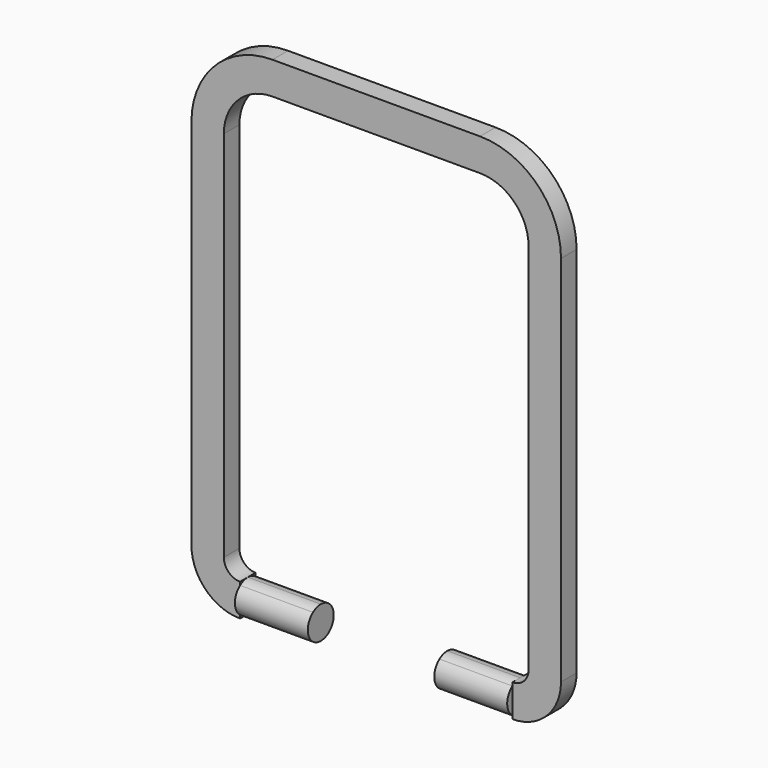
from build123d import *
from build123d import SkipClean  # not in build123d's __all__

# Parameters (mm, degrees)
F1_DEPTH = 1.2
F3_DEPTH = 4.5
F4_DEPTH = 4.5
F6_DEPTH = 4.5
F7_DEPTH = 4.5


with BuildPart() as f1:
    # F0 (on Front) → F1 (new body)
    with BuildSketch(Plane.XZ):
        with BuildLine():
            Line((5.55, 0), (-7.25, 0))
            ThreePointArc((-7.25, 0), (-10.7855339059, -1.4644660941), (-12.25, -5))
            Line((-12.25, -5), (-12.25, -28))
            ThreePointArc((-12.25, -28), (-11.3713203436, -30.1213203436), (-9.25, -31))
            Line((-9.25, -31), (-4.75, -31))
            Line((-4.75, -31), (-4.75, -29))
            Line((-4.75, -29), (-9.25, -29))
            ThreePointArc((-9.25, -29), (-9.9571067812, -28.7071067812), (-10.25, -28))
            Line((-10.25, -28), (-10.25, -5))
            ThreePointArc((-10.25, -5), (-9.3713203436, -2.8786796564), (-7.25, -2))
            Line((-7.25, -2), (5.55, -2))
            ThreePointArc((5.55, -2), (7.6713203436, -2.8786796564), (8.55, -5))
            Line((8.55, -5), (8.55, -28))
            ThreePointArc((8.55, -28), (8.2571067812, -28.7071067812), (7.55, -29))
            Line((7.55, -29), (3.05, -29))
            Line((3.05, -29), (3.05, -31))
            Line((3.05, -31), (7.55, -31))
            ThreePointArc((7.55, -31), (9.6713203436, -30.1213203436), (10.55, -28))
            Line((10.55, -28), (10.55, -5))
            ThreePointArc((10.55, -5), (9.0855339059, -1.4644660941), (5.55, 0))
        make_face()
    extrude(amount=F1_DEPTH)

    # F2 (on face) → F3 (join)
    with BuildSketch(Plane.YZ.offset(-4.75)):
        with BuildLine():
            Line((-1.2, -30.8), (-1.2, -29.2))
            ThreePointArc((-1.2, -29.2), (-1.6, -30), (-1.2, -30.8))
        make_face()
        with BuildLine():
            ThreePointArc((-0.6, -29), (-0.916227766, -29.0513167019), (-1.2, -29.2))
            Line((-1.2, -29.2), (-1.2, -30.8))
            ThreePointArc((-1.2, -30.8), (-0.916227766, -30.9486832981), (-0.6, -31))
            ThreePointArc((-0.6, -31), (-0.283772234, -30.9486832981), (0, -30.8))
            Line((0, -30.8), (0, -29.2))
            ThreePointArc((0, -29.2), (-0.283772234, -29.0513167019), (-0.6, -29))
        make_face()
        with BuildLine():
            ThreePointArc((0.4, -30), (0.294427191, -29.5527864045), (0, -29.2))
            Line((0, -29.2), (0, -30.8))
            ThreePointArc((0, -30.8), (0.294427191, -30.4472135955), (0.4, -30))
        make_face()
    extrude(amount=-F3_DEPTH)

    # F2 (on face) → F4 (cut)
    with BuildSketch(Plane.YZ.offset(-4.75)):
        with BuildLine():
            Line((0, -29), (-0.6, -29))
            ThreePointArc((-0.6, -29), (-0.283772234, -29.0513167019), (0, -29.2))
            Line((0, -29.2), (0, -29))
        make_face()
        with BuildLine():
            Line((-0.6, -29), (-1.2, -29))
            Line((-1.2, -29), (-1.2, -29.2))
            ThreePointArc((-1.2, -29.2), (-0.916227766, -29.0513167019), (-0.6, -29))
        make_face()
        with BuildLine():
            ThreePointArc((0, -30.8), (-0.283772234, -30.9486832981), (-0.6, -31))
            Line((-0.6, -31), (0, -31))
            Line((0, -31), (0, -30.8))
        make_face()
        with BuildLine():
            ThreePointArc((-0.6, -31), (-0.916227766, -30.9486832981), (-1.2, -30.8))
            Line((-1.2, -30.8), (-1.2, -31))
            Line((-1.2, -31), (-0.6, -31))
        make_face()
    with SkipClean():  # cleaning this boolean's faces spoils the solid; the shape is the same uncleaned
        extrude(amount=-F4_DEPTH, mode=Mode.SUBTRACT)

    # F5 (on face) → F6 (join)
    with BuildSketch(Plane(origin=(3.05, 0, 0), x_dir=(0, -1, 0), z_dir=(-1, 0, 0))):
        with BuildLine():
            Line((1.2, -30.8), (1.2, -29.2))
            ThreePointArc((1.2, -29.2), (0.916227766, -29.0513167019), (0.6, -29))
            ThreePointArc((0.6, -29), (0.283772234, -29.0513167019), (0, -29.2))
            Line((0, -29.2), (0, -30.8))
            ThreePointArc((0, -30.8), (0.283772234, -30.9486832981), (0.6, -31))
            ThreePointArc((0.6, -31), (0.916227766, -30.9486832981), (1.2, -30.8))
        make_face()
        with BuildLine():
            Line((0, -30.8), (0, -29.2))
            ThreePointArc((0, -29.2), (-0.4, -30), (0, -30.8))
        make_face()
        with BuildLine():
            ThreePointArc((1.6, -30), (1.494427191, -29.5527864045), (1.2, -29.2))
            Line((1.2, -29.2), (1.2, -30.8))
            ThreePointArc((1.2, -30.8), (1.494427191, -30.4472135955), (1.6, -30))
        make_face()
    extrude(amount=-F6_DEPTH)

    # F5 (on face) → F7 (cut)
    with BuildSketch(Plane(origin=(3.05, 0, 0), x_dir=(0, -1, 0), z_dir=(-1, 0, 0))):
        with BuildLine():
            ThreePointArc((0, -29.2), (0.283772234, -29.0513167019), (0.6, -29))
            Line((0.6, -29), (0, -29))
            Line((0, -29), (0, -29.2))
        make_face()
        with BuildLine():
            Line((1.2, -29.2), (1.2, -29))
            Line((1.2, -29), (0.6, -29))
            ThreePointArc((0.6, -29), (0.916227766, -29.0513167019), (1.2, -29.2))
        make_face()
        with BuildLine():
            Line((0, -31), (0.6, -31))
            ThreePointArc((0.6, -31), (0.283772234, -30.9486832981), (0, -30.8))
            Line((0, -30.8), (0, -31))
        make_face()
        with BuildLine():
            Line((1.2, -31), (1.2, -30.8))
            ThreePointArc((1.2, -30.8), (0.916227766, -30.9486832981), (0.6, -31))
            Line((0.6, -31), (1.2, -31))
        make_face()
    with SkipClean():  # cleaning this boolean's faces spoils the solid; the shape is the same uncleaned
        extrude(amount=-F7_DEPTH, mode=Mode.SUBTRACT)


solid = f1.part
